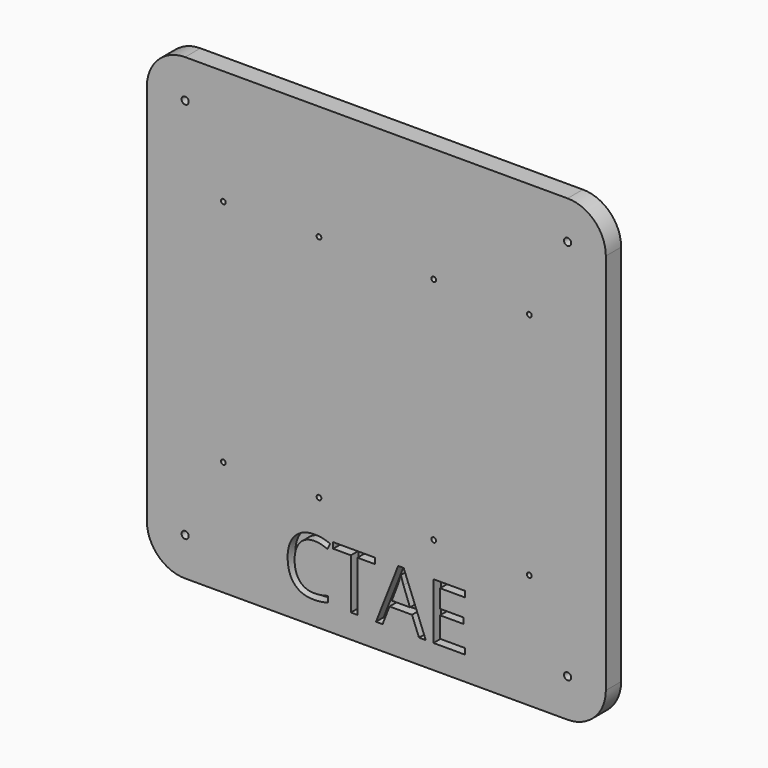
from build123d import *

# Parameters (mm, degrees)
F1_DEPTH     = 12.7
F2_D         = 4.7752
F3_D         = 3.175
F4_TEXT_SIZE = 52.2463888889
F5_DEPTH     = 6.35


# Not quite as in the source:
# - Text() gives the source's letters only with a copy of the font that has no kerning and outlines rounded to 1/6400 em; it was checked with that copy


with BuildPart() as f1:
    # F0 (on Front) → F1 (new body)
    with BuildSketch(Plane.XZ):
        with BuildLine():
            ThreePointArc((0, 25.4), (7.4394877579, 7.4394877579), (25.4, 0))
            Line((25.4, 0), (279.4, 0))
            ThreePointArc((279.4, 0), (297.3605122421, 7.4394877579), (304.8, 25.4))
            Line((304.8, 25.4), (304.8, 279.4))
            ThreePointArc((304.8, 279.4), (297.3605122421, 297.3605122421), (279.4, 304.8))
            Line((279.4, 304.8), (25.4, 304.8))
            ThreePointArc((25.4, 304.8), (7.4394877579, 297.3605122421), (0, 279.4))
            Line((0, 279.4), (0, 25.4))
        make_face()
    extrude(amount=F1_DEPTH)

    # F2 (through all)
    with Locations(Plane(origin=(0, 0, 0), x_dir=(1, 0, 0), z_dir=(0, 1, 0))):
        with Locations((25.4, -279.4), (25.4, -25.4), (279.4, -25.4), (279.4, -279.4)):
            Hole(F2_D / 2)

    # F3 (through all)
    with Locations(Plane(origin=(0, 0, 0), x_dir=(1, 0, 0), z_dir=(0, 1, 0))):
        with Locations((50.8, -228.6), (114.3, -228.6), (190.5, -228.6), (254, -228.6), (254, -76.2), (190.5, -76.2), (50.8, -76.2), (114.3, -76.2)):
            Hole(F3_D / 2)

    # F4 (on face) → F5 (cut)
    with BuildSketch(Plane.XZ.offset(12.7)):
        with Locations((90.2798599609, 15.9004)):
            Text('CTAE', F4_TEXT_SIZE, font='Open Sans', text_align=(TextAlign.LEFT, TextAlign.BOTTOM))
    extrude(amount=-F5_DEPTH, mode=Mode.SUBTRACT)


solid = f1.part
